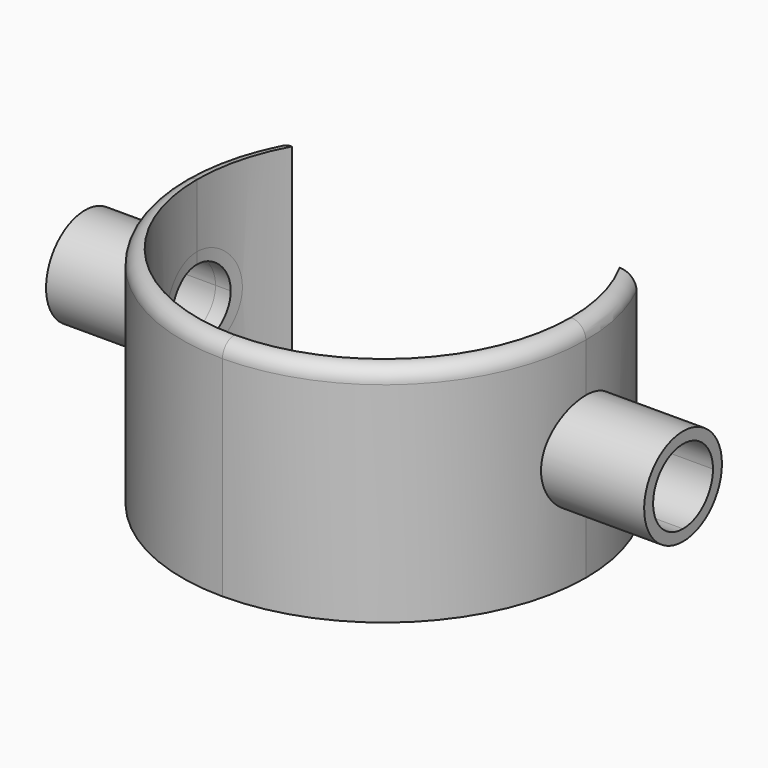
from build123d import *
from build123d import SkipClean  # not in build123d's __all__

# Parameters (mm, degrees)
F1_DEPTH = 30
F3_DEPTH = 40
F4_DEPTH = 25
F5_DEPTH = 30
F7_R     = 1.99999


# Not quite as in the source:
# - a fillet or chamfer is up to 0.001 mm smaller than in the source, because OpenCascade refuses the exact size


with BuildPart() as f1:
    # F0 (on Top) → F1 (new body)
    with BuildSketch(Plane.XY):
        with BuildLine():
            ThreePointArc((25, 0), (17.6776695297, -17.6776695297), (0, -25))
            Line((0, -25), (0, -27))
            ThreePointArc((0, -27), (19.091883092, -19.091883092), (27, 0))
            ThreePointArc((27, 0), (26.2872866383, 6.1626748408), (24.1867732449, 12))
            Line((24.1867732449, 12), (21.9317121995, 12))
            ThreePointArc((21.9317121995, 12), (24.2207845144, 6.1930281371), (25, 0))
        make_face()
    extrude(amount=F1_DEPTH)

    # F2 (on Right) → F3 (join)
    with BuildSketch(Plane.YZ):
        with BuildLine():
            ThreePointArc((6.5, 15), (-4.5961940777, 19.5961940777), (0, 8.5))
            ThreePointArc((0, 8.5), (4.5961940777, 10.4038059223), (6.5, 15))
        make_face()
        with BuildLine():
            ThreePointArc((5, 15), (3.5355339059, 11.4644660941), (0, 10))
            ThreePointArc((0, 10), (-3.5355339059, 18.5355339059), (5, 15))
        make_face(mode=Mode.SUBTRACT)
    extrude(amount=F3_DEPTH)

    # F0 (on Top) → F4 (cut)
    with BuildSketch(Plane.XY):
        with BuildLine():
            Line((0, 0), (0, -25))
            ThreePointArc((0, -25), (17.6776695297, -17.6776695297), (25, 0))
            ThreePointArc((25, 0), (24.2207845144, 6.1930281371), (21.9317121995, 12))
            Line((21.9317121995, 12), (0, 12))
            Line((0, 12), (0, 0))
        make_face()
    extrude(amount=F4_DEPTH, mode=Mode.SUBTRACT)

    # F2 (on Right) → F5 (cut)
    with BuildSketch(Plane.YZ):
        with BuildLine():
            ThreePointArc((5, 15), (-3.5355339059, 18.5355339059), (0, 10))
            ThreePointArc((0, 10), (3.5355339059, 11.4644660941), (5, 15))
        make_face()
    extrude(amount=F5_DEPTH, mode=Mode.SUBTRACT)

    # F6: F1 across plane


with BuildPart() as f1_1:
    add(f1.part, clean=False)
    with SkipClean():  # cleaning this boolean's faces spoils the solid; the shape is the same uncleaned
        add(f1.part.mirror(Plane.YZ), clean=False)

    # F7 (radius 2 in the source; OpenCascade refuses exactly that, so slightly less here)
    f7_edges = [f1_1.edges().sort_by_distance(p)[0] for p in [
        (-22.945588, -14.230249, 30),
        (22.945588, -14.230249, 30),
    ]]
    fillet(f7_edges, radius=F7_R)


solid = f1_1.part
